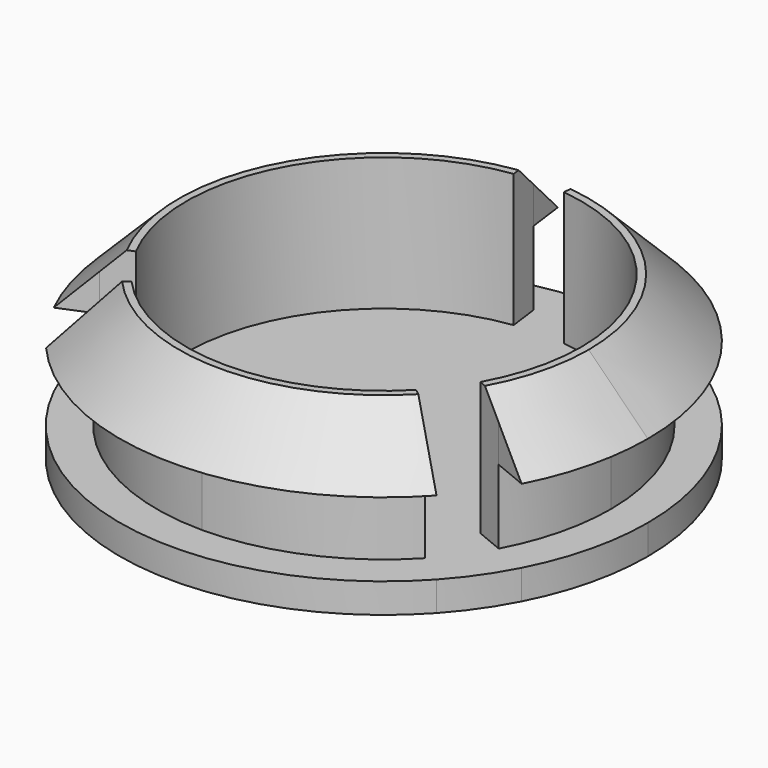
from build123d import *

# Parameters (mm, degrees)
F1_DEPTH = 1
F2_DEPTH = 5.5
F3_START = 3.5
F3_DEPTH = 2
F4_SIZE  = 1.99999


# Not quite as in the source:
# - a fillet or chamfer is up to 0.001 mm smaller than in the source, because OpenCascade refuses the exact size


with BuildPart() as f1:
    # F0 (on Top) → F1 (new body)
    with BuildSketch(Plane.XY):
        with BuildLine():
            ThreePointArc((6.675, 0), (4.9879380463, 4.4357749094), (0.7795396115, 6.6293244749))
            ThreePointArc((0.7795396115, 6.6293244749), (-0.0613991479, 6.6747176079), (-0.9013605528, 6.6138622721))
            ThreePointArc((-0.9013605528, 6.6138622721), (-5.9267464923, 3.0707166942), (-5.9228974074, -3.0781343864))
            ThreePointArc((-5.9228974074, -3.0781343864), (-5.4750931221, -3.8182430914), (-4.9353373694, -4.4942263016))
            ThreePointArc((-4.9353373694, -4.4942263016), (-2.6978384344, -6.1055133103), (0, -6.675))
            ThreePointArc((0, -6.675), (2.6066720123, -6.1449886916), (4.7993917719, -4.6391231521))
            ThreePointArc((4.7993917719, -4.6391231521), (5.3679142179, -3.9675082796), (5.8431534535, -3.2269463459))
            ThreePointArc((5.8431534535, -3.2269463459), (6.4636937699, -1.6662196281), (6.675, 0))
        make_face()
        with BuildLine():
            Line((-5.9228974074, -3.0781343864), (-6.849796149, -3.4620684161))
            ThreePointArc((-6.849796149, -3.4620684161), (-6.3438696558, -4.3198313381), (-5.7311395238, -5.1048667718))
            Line((-5.7311395238, -5.1048667718), (-4.9353373694, -4.4942263016))
            ThreePointArc((-4.9353373694, -4.4942263016), (-5.4750931221, -3.8182430914), (-5.9228974074, -3.0781343864))
        make_face()
        with BuildLine():
            Line((-6.849796149, -3.4620684161), (-8.0074646458, -3.9415904082))
            ThreePointArc((-8.0074646458, -3.9415904082), (-7.4289702623, -4.9463143695), (-6.7251178515, -5.8675731681))
            Line((-6.7251178515, -5.8675731681), (-5.7311395238, -5.1048667718))
            ThreePointArc((-5.7311395238, -5.1048667718), (-6.3438696558, -4.3198313381), (-6.849796149, -3.4620684161))
        make_face()
        with BuildLine():
            Line((0.9100766885, 7.6208520141), (1.0732446043, 8.8602353817))
            ThreePointArc((1.0732446043, 8.8602353817), (-0.0613988555, 8.9247888031), (-1.1950467583, 8.8446304754))
            Line((-1.1950467583, 8.8446304754), (-1.0318879198, 7.6053160566))
            ThreePointArc((-1.0318879198, 7.6053160566), (-0.0613989862, 7.6747544042), (0.9100766885, 7.6208520141))
        make_face()
        with BuildLine():
            Line((-1.0318879198, 7.6053160566), (-1.1950467583, 8.8446304754))
            ThreePointArc((-1.1950467583, 8.8446304754), (-7.8767642568, 4.196690344), (-8.0074646458, -3.9415904082))
            Line((-8.0074646458, -3.9415904082), (-6.849796149, -3.4620684161))
            ThreePointArc((-6.849796149, -3.4620684161), (-6.7935252783, 3.5712237809), (-1.0318879198, 7.6053160566))
        make_face()
        with BuildLine():
            ThreePointArc((-6.7251178515, -5.8675731681), (-3.6937470456, -8.1247681667), (0, -8.925))
            Line((0, -8.925), (0, -7.675))
            ThreePointArc((0, -7.675), (-3.1405232467, -7.0030521015), (-5.7311395238, -5.1048667718))
            Line((-5.7311395238, -5.1048667718), (-6.7251178515, -5.8675731681))
        make_face()
        with BuildLine():
            ThreePointArc((0, -8.925), (3.6032793864, -8.1652925645), (6.5931272563, -6.0155047986))
            Line((6.5931272563, -6.0155047986), (5.597241272, -5.2513346059))
            ThreePointArc((5.597241272, -5.2513346059), (3.0497239137, -7.043068156), (0, -7.675))
            Line((0, -7.675), (0, -8.925))
        make_face()
        with BuildLine():
            ThreePointArc((6.5931272563, -6.0155047986), (7.3257881446, -5.0978871172), (7.9316419101, -4.0920265895))
            Line((7.9316419101, -4.0920265895), (6.7720820443, -3.6117211667))
            ThreePointArc((6.7720820443, -3.6117211667), (6.2387597231, -4.4702910551), (5.597241272, -5.2513346059))
            Line((5.597241272, -5.2513346059), (6.5931272563, -6.0155047986))
        make_face()
        with BuildLine():
            ThreePointArc((7.9316419101, -4.0920265895), (8.6731058176, -2.1054359349), (8.925, 0))
            ThreePointArc((8.925, 0), (6.679608263, 5.9193292233), (1.0732446043, 8.8602353817))
            Line((1.0732446043, 8.8602353817), (0.9100766885, 7.6208520141))
            ThreePointArc((0.9100766885, 7.6208520141), (5.7397937064, 5.0951342679), (7.675, 0))
            ThreePointArc((7.675, 0), (7.4458496725, -1.8614369866), (6.7720820443, -3.6117211667))
            Line((6.7720820443, -3.6117211667), (7.9316419101, -4.0920265895))
        make_face()
        with BuildLine():
            ThreePointArc((5.597241272, -5.2513346059), (6.2387597231, -4.4702910551), (6.7720820443, -3.6117211667))
            Line((6.7720820443, -3.6117211667), (5.8431534535, -3.2269463459))
            ThreePointArc((5.8431534535, -3.2269463459), (5.3679142179, -3.9675082796), (4.7993917719, -4.6391231521))
            Line((4.7993917719, -4.6391231521), (5.597241272, -5.2513346059))
        make_face()
        with BuildLine():
            Line((0.7795396115, 6.6293244749), (0.9100766885, 7.6208520141))
            ThreePointArc((0.9100766885, 7.6208520141), (-0.0613989862, 7.6747544042), (-1.0318879198, 7.6053160566))
            Line((-1.0318879198, 7.6053160566), (-0.9013605528, 6.6138622721))
            ThreePointArc((-0.9013605528, 6.6138622721), (-0.0613991479, 6.6747176079), (0.7795396115, 6.6293244749))
        make_face()
    extrude(amount=F1_DEPTH)

    # F0 (on Top) → F2 (join)
    with BuildSketch(Plane.XY):
        with BuildLine():
            Line((-0.9013605528, 6.6138622721), (-1.0318879198, 7.6053160566))
            ThreePointArc((-1.0318879198, 7.6053160566), (-6.7935252783, 3.5712237809), (-6.849796149, -3.4620684161))
            Line((-6.849796149, -3.4620684161), (-5.9228974074, -3.0781343864))
            ThreePointArc((-5.9228974074, -3.0781343864), (-5.9267464923, 3.0707166942), (-0.9013605528, 6.6138622721))
        make_face()
        with BuildLine():
            ThreePointArc((7.675, 0), (5.7397937064, 5.0951342679), (0.9100766885, 7.6208520141))
            Line((0.9100766885, 7.6208520141), (0.7795396115, 6.6293244749))
            ThreePointArc((0.7795396115, 6.6293244749), (4.9879380463, 4.4357749094), (6.675, 0))
            ThreePointArc((6.675, 0), (6.4636937699, -1.6662196281), (5.8431534535, -3.2269463459))
            Line((5.8431534535, -3.2269463459), (6.7720820443, -3.6117211667))
            ThreePointArc((6.7720820443, -3.6117211667), (7.4458496725, -1.8614369866), (7.675, 0))
        make_face()
        with BuildLine():
            ThreePointArc((-5.7311395238, -5.1048667718), (-3.1405232467, -7.0030521015), (0, -7.675))
            Line((0, -7.675), (0, -6.675))
            ThreePointArc((0, -6.675), (-2.6978384344, -6.1055133103), (-4.9353373694, -4.4942263016))
            Line((-4.9353373694, -4.4942263016), (-5.7311395238, -5.1048667718))
        make_face()
        with BuildLine():
            ThreePointArc((0, -7.675), (3.0497239137, -7.043068156), (5.597241272, -5.2513346059))
            Line((5.597241272, -5.2513346059), (4.7993917719, -4.6391231521))
            ThreePointArc((4.7993917719, -4.6391231521), (2.6066720123, -6.1449886916), (0, -6.675))
            Line((0, -6.675), (0, -7.675))
        make_face()
    extrude(amount=F2_DEPTH)

    # F0 (on Top) → F3 (join)
    with BuildSketch(Plane.XY.offset(F3_START)):
        with BuildLine():
            Line((-1.0318879198, 7.6053160566), (-1.1950467583, 8.8446304754))
            ThreePointArc((-1.1950467583, 8.8446304754), (-7.8767642568, 4.196690344), (-8.0074646458, -3.9415904082))
            Line((-8.0074646458, -3.9415904082), (-6.849796149, -3.4620684161))
            ThreePointArc((-6.849796149, -3.4620684161), (-6.7935252783, 3.5712237809), (-1.0318879198, 7.6053160566))
        make_face()
        with BuildLine():
            ThreePointArc((7.9316419101, -4.0920265895), (8.6731058176, -2.1054359349), (8.925, 0))
            ThreePointArc((8.925, 0), (6.679608263, 5.9193292233), (1.0732446043, 8.8602353817))
            Line((1.0732446043, 8.8602353817), (0.9100766885, 7.6208520141))
            ThreePointArc((0.9100766885, 7.6208520141), (5.7397937064, 5.0951342679), (7.675, 0))
            ThreePointArc((7.675, 0), (7.4458496725, -1.8614369866), (6.7720820443, -3.6117211667))
            Line((6.7720820443, -3.6117211667), (7.9316419101, -4.0920265895))
        make_face()
        with BuildLine():
            ThreePointArc((0, -8.925), (3.6032793864, -8.1652925645), (6.5931272563, -6.0155047986))
            Line((6.5931272563, -6.0155047986), (5.597241272, -5.2513346059))
            ThreePointArc((5.597241272, -5.2513346059), (3.0497239137, -7.043068156), (0, -7.675))
            Line((0, -7.675), (0, -8.925))
        make_face()
        with BuildLine():
            ThreePointArc((-6.7251178515, -5.8675731681), (-3.6937470456, -8.1247681667), (0, -8.925))
            Line((0, -8.925), (0, -7.675))
            ThreePointArc((0, -7.675), (-3.1405232467, -7.0030521015), (-5.7311395238, -5.1048667718))
            Line((-5.7311395238, -5.1048667718), (-6.7251178515, -5.8675731681))
        make_face()
    extrude(amount=F3_DEPTH)

    # F4 (size 2 in the source; OpenCascade refuses exactly that, so slightly less here)
    f4_edges = [f1.edges().sort_by_distance(p)[0] for p in [
        (-7.876764, 4.19669, 5.5),
        (-0.099128, -8.924449, 5.5),
        (7.887475, 4.176525, 5.5),
    ]]
    chamfer(f4_edges, length=F4_SIZE)


solid = f1.part
